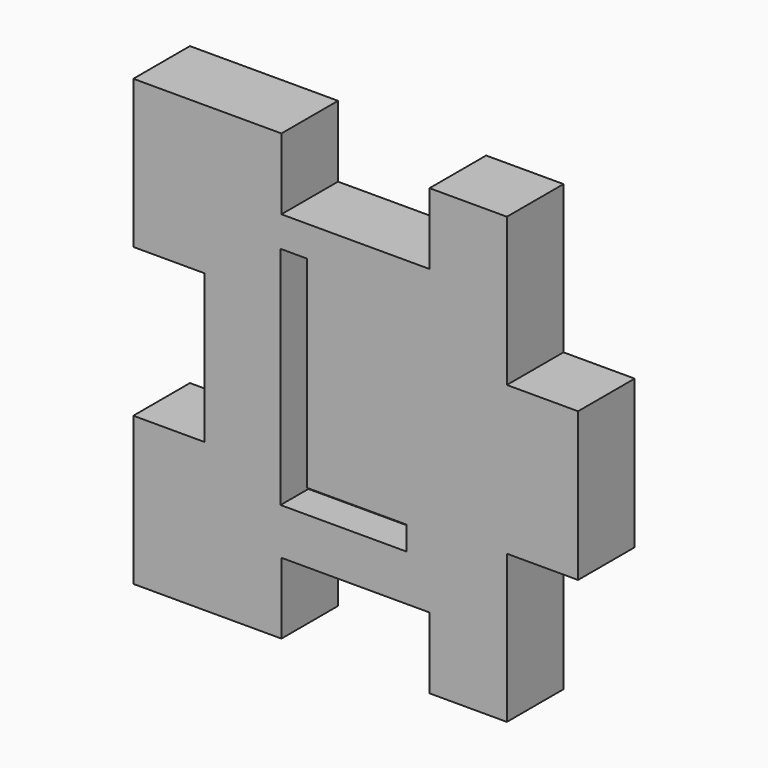
from build123d import *

# Parameters (mm, degrees)
F1_DEPTH     = 2.032
F2_TEXT_SIZE = 9.076394429
F3_DEPTH     = 1


# Not quite as in the source:
# - a length typed as a fraction of an inch, garbled in the dataset ("3 / 203.2 mm" for 3/8 in), is restored
# - Text() gives the source's letters only with a copy of the font that has no kerning and outlines rounded to 1/6400 em; it was checked with that copy


with BuildPart() as f1:
    # F0 (on Front) → F1 (new body)
    with BuildSketch(Plane.XZ):
        Polygon((-10.9897290399, 29.0234165891), (-10.9897290399, 26.8898165891), (-10.9897290399, 24.7562165891), (-13.0344290399, 24.7562165891), (-13.0344290399, 20.5017165891), (-8.7799290399, 20.5017165891), (-8.7799290399, 22.5464165891), (-4.5254290399, 22.5464165891), (-4.5254290399, 20.5017165891), (-2.3029290399, 20.5017165891), (-2.3029290399, 24.7562165891), (-0.2582290399, 24.7562165891), (-0.2582290399, 29.0234165891), (-2.3029290399, 29.0234165891), (-2.3029290399, 33.2779165891), (-4.5254290399, 33.2779165891), (-4.5254290399, 31.2332165891), (-8.7799290399, 31.2332165891), (-8.7799290399, 33.2779165891), (-13.0344290399, 33.2779165891), (-13.0344290399, 29.0234165891), align=None)
    extrude(amount=F1_DEPTH)

    # F2 (on face) → F3 (cut)
    with BuildSketch(Plane.XZ.offset(2.032)):
        with Locations((-9.6958548804, 23.8721947685)):
            Text('L', F2_TEXT_SIZE, font='Open Sans', text_align=(TextAlign.LEFT, TextAlign.BOTTOM))
    extrude(amount=-F3_DEPTH, mode=Mode.SUBTRACT)


solid = f1.part
